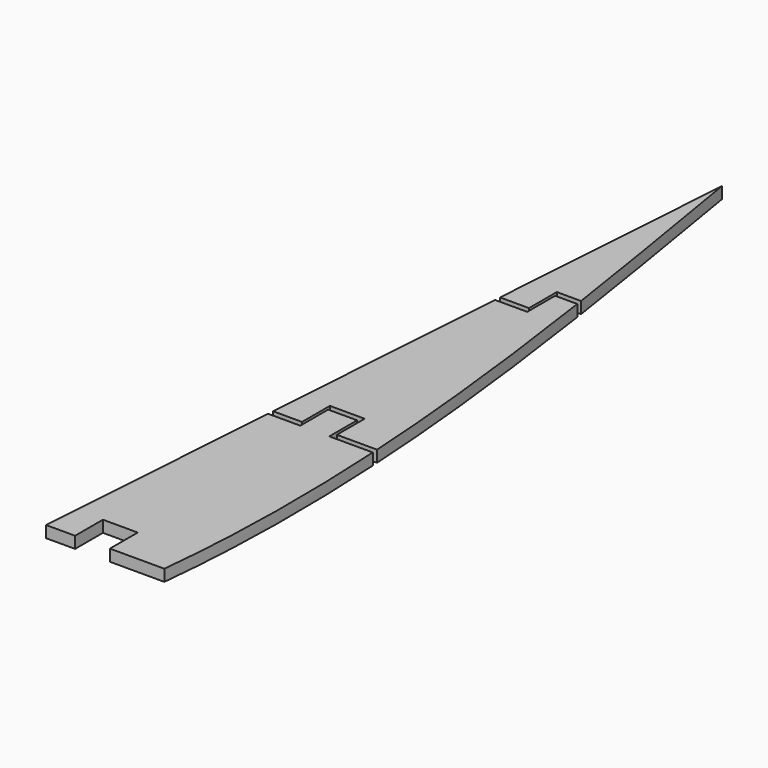
from build123d import *

# Parameters (mm, degrees)
F1_DEPTH = 2


with BuildPart() as f1:
    # F0 (on Top) → F1 (new body)
    with BuildSketch(Plane.XY):
        with BuildLine():
            add(Edge.make_bspline(
                [(-34.4950757243, 25.2946874197), (-31.9979345744, 8.3570934049), (-29.9651182209, -8.3919319955), (-29.0050185061, -24.7053125803)],
                knots=[0.1484687426, 0.1484687426, 0.1484687426, 0.1484687426, 0.343003199, 0.343003199, 0.343003199, 0.343003199], degree=3))
            Line((-34.4950757243, 25.2946874197), (-38.3131276168, 25.2946874197))
            Line((-38.3131276168, 25.2946874197), (-38.3131276168, 19.2946874197))
            Line((-38.3131276168, 19.2946874197), (-43.8826658205, 19.2946874197))
            Line((-43.8826658205, 19.2946874197), (-46.9423467859, -24.7053125803))
            Line((-46.9423467859, -24.7053125803), (-41.9423467859, -24.7053125803))
            Line((-41.9423467859, -24.7053125803), (-41.9423467859, -18.7053125803))
            Line((-41.9423467859, -18.7053125803), (-35.9423467859, -18.7053125803))
            Line((-35.9423467859, -18.7053125803), (-35.9423467859, -24.7053125803))
            Line((-35.9423467859, -24.7053125803), (-29.0050185061, -24.7053125803))
        make_face()
    extrude(amount=F1_DEPTH)


with BuildPart() as f1b:
    # F0 (on Top) → F1, piece 2 (new body)
    with BuildSketch(Plane.XY):
        with BuildLine():
            add(Edge.make_bspline(
                [(-40.7534466514, 64.2946874197), (-38.6332764023, 51.5941678927), (-36.5131061532, 38.8936483656), (-34.6430102214, 26.2946874197)],
                knots=[0, 0, 0, 0, 0.1446411187, 0.1446411187, 0.1446411187, 0.1446411187], degree=3))
            Line((-40.7534466514, 64.2946874197), (-43.8131276168, 20.2946874197))
            Line((-43.8131276168, 20.2946874197), (-38.8131276168, 20.2946874197))
            Line((-38.8131276168, 20.2946874197), (-38.8131276168, 26.2946874197))
            Line((-38.8131276168, 26.2946874197), (-34.6430102214, 26.2946874197))
        make_face()
    extrude(amount=F1_DEPTH)


with BuildPart() as f1c:
    # F0 (on Top) → F1, piece 3 (new body)
    with BuildSketch(Plane.XY):
        with BuildLine():
            add(Edge.make_bspline(
                [(-28.9474830129, -25.7053125803), (-28.0980614593, -40.8166316864), (-28.1818146304, -55.548975846), (-29.6839084476, -69.7053125803)],
                knots=[0.3469803254, 0.3469803254, 0.3469803254, 0.3469803254, 0.5273785134, 0.5273785134, 0.5273785134, 0.5273785134], degree=3))
            Line((-28.9474830129, -25.7053125803), (-36.4423467859, -25.7053125803))
            Line((-36.4423467859, -25.7053125803), (-36.4423467859, -19.7053125803))
            Line((-36.4423467859, -19.7053125803), (-41.4423467859, -19.7053125803))
            Line((-41.4423467859, -19.7053125803), (-41.4423467859, -25.7053125803))
            Line((-41.4423467859, -25.7053125803), (-47.0118849897, -25.7053125803))
            Line((-47.0118849897, -25.7053125803), (-50.0715659551, -69.7053125803))
            Line((-50.0715659551, -69.7053125803), (-45.0715659551, -69.7053125803))
            Line((-45.0715659551, -69.7053125803), (-45.0715659551, -63.7053125803))
            Line((-45.0715659551, -63.7053125803), (-39.0715659551, -63.7053125803))
            Line((-39.0715659551, -63.7053125803), (-39.0715659551, -69.7053125803))
            Line((-39.0715659551, -69.7053125803), (-29.6839084476, -69.7053125803))
        make_face()
    extrude(amount=F1_DEPTH)


solid = Compound([f1.part, f1b.part, f1c.part])
